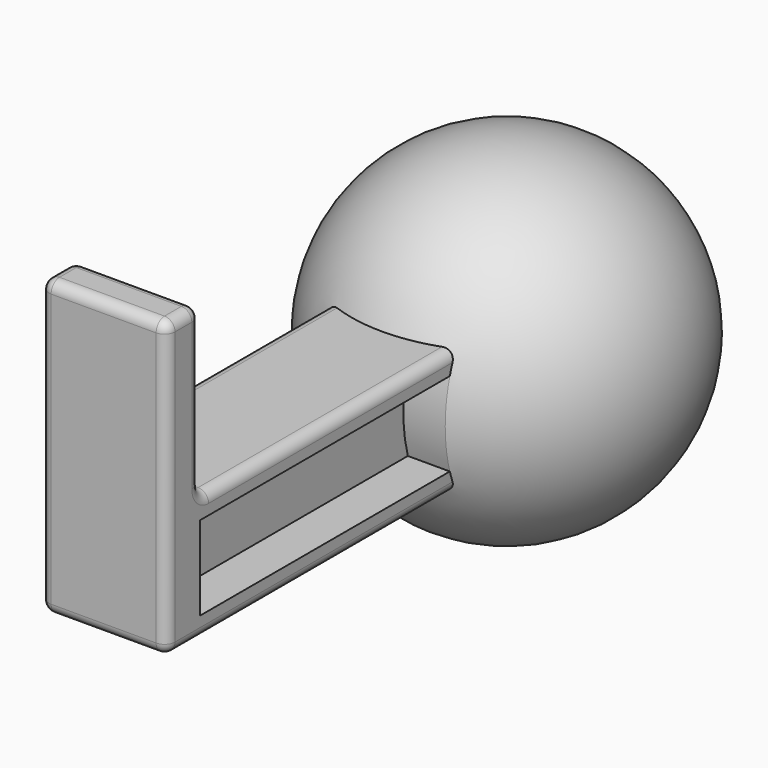
from build123d import *

# Parameters (mm, degrees)
F2_W     = 19.05
F2_H     = 19.05
F3_DEPTH = 76.2
F4_W     = 19.05
F4_H     = 6.35
F5_DEPTH = 25.4
F7_DEPTH = 6.35
F10_F1_R = 1.5875
F10_F2_R = 1.5875


with BuildPart() as f1:
    # F0 (on Top) → F1 (revolve)
    with BuildSketch(Plane.XY):
        with BuildLine():
            Line((0, -25.4), (0, 25.4))
            ThreePointArc((0, 25.4), (-25.4, 0), (0, -25.4))
        make_face()
    revolve(axis=Axis((0, -0.8307937533, 0), (0, 1, 0)))

    # F2 (on Front) → F3 (join)
    with BuildSketch(Plane.XZ):
        Rectangle(F2_W, F2_H)
    extrude(amount=F3_DEPTH)

    # F4 (on face) → F5 (join)
    with BuildSketch(Plane.XY.offset(9.525)):
        with Locations((0, -73.025)):
            Rectangle(F4_W, F4_H)
    extrude(amount=F5_DEPTH)


with BuildPart() as f7:
    # F6 (on face) → F7 (new body, symmetric)
    with BuildSketch(Plane.YZ.offset(9.525)):
        with BuildLine():
            Line((-22.6740352606, 6.35), (-69.85, 6.35))
            Line((-69.85, 6.35), (-69.85, -6.35))
            Line((-69.85, -6.35), (-22.6740352606, -6.35))
            ThreePointArc((-22.6740352606, -6.35), (-23.5464301965, 0), (-22.6740352606, 6.35))
        make_face()
    extrude(amount=F7_DEPTH, both=True)


with BuildPart() as f8_1:
    # F8: instance of F7
    add(f7.part.mirror(Plane.YZ))


with BuildPart() as f1_1:
    add(f1.part)

    # F9: cut F8_1, F7
    add(f8_1.part, mode=Mode.SUBTRACT)
    add(f7.part, mode=Mode.SUBTRACT)

    # F10: fillet of radius 1.5875 on 12 edges, made by hand

    # F10_f1
    f10_f1_edges = [f1_1.edges().sort_by_distance(p)[0] for p in [
        (0, -69.85, 9.525),
    ]]
    fillet(f10_f1_edges, radius=F10_F1_R)

    # F10_f2
    f10_f2_edges = [f1_1.edges().sort_by_distance(p)[0] for p in [
        (0, -76.2, 34.925),
        (9.525, -73.025, 34.925),
        (0, -69.85, 34.925),
        (-9.525, -73.025, 34.925),
        (9.525, -76.2, 12.7),
        (-9.525, -76.2, 12.7),
        (-9.525, -69.85, 23.01875),
        (9.525, -69.85, 23.01875),
        (0, -76.2, -9.525),
        (9.525, -48.8669488482, -9.525),
        (-9.525, -48.8669488482, -9.525),
        (9.525, -69.3850320151, 9.9899679849),
        (-9.525, -69.3850320151, 9.9899679849),
    ]]
    fillet(f10_f2_edges, radius=F10_F2_R)


solid = f1_1.part
